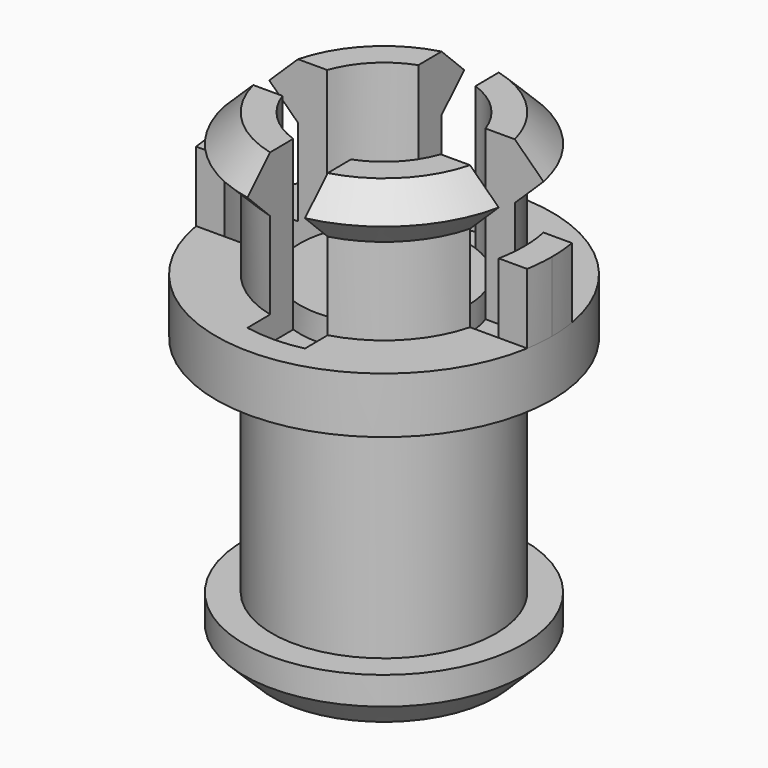
from build123d import *

# Parameters (mm, degrees)
F0_R      = 5
F1_DEPTH  = 2
F2_R      = 4
F3_DEPTH  = 8
F4_R      = 6
F5_DEPTH  = 2
F7_DEPTH  = 2.5
F10_DEPTH = 8
F11_SIZE  = 1
F8_R      = 4
F8_R_2    = 3
F12_DEPTH = 3.1
F13_R     = 5
F13_R_2   = 4
F13_R_3   = 3
F14_DEPTH = 2
F16_DEPTH = 6
F17_SIZE  = 0.99999


# Not quite as in the source:
# - a fillet or chamfer is up to 0.001 mm smaller than in the source, because OpenCascade refuses the exact size


with BuildPart() as f1:
    # F0 (on Top) → F1 (new body)
    with BuildSketch(Plane.XY):
        Circle(F0_R)
    extrude(amount=F1_DEPTH)

    # F2 (on face) → F3 (join)
    with BuildSketch(Plane.XY.offset(2)):
        Circle(F2_R)
    extrude(amount=F3_DEPTH)

    # F4 (on face) → F5 (join)
    with BuildSketch(Plane.XY.offset(10)):
        Circle(F4_R)
    extrude(amount=F5_DEPTH)

    # F6 (on face) → F7 (join)
    with BuildSketch(Plane.XY.offset(12)):
        with BuildLine():
            ThreePointArc((6, 0), (5.9789831367, 0.5017575617), (5.9160797831, 1))
            Line((5.9160797831, 1), (4.5160797831, 1))
            Line((4.5160797831, 1), (4.5160797831, -1))
            Line((4.5160797831, -1), (5.9160797831, -1))
            ThreePointArc((5.9160797831, -1), (5.9789831367, -0.5017575617), (6, 0))
        make_face()
        with BuildLine():
            Line((-4.5160797831, 1), (-5.9160797831, 1))
            ThreePointArc((-5.9160797831, 1), (-6, 0), (-5.9160797831, -1))
            Line((-5.9160797831, -1), (-4.5160797831, -1))
            Line((-4.5160797831, -1), (-4.5160797831, 1))
        make_face()
    extrude(amount=F7_DEPTH)

    # F9 (on face) → F10 (cut)
    with BuildSketch(Plane(origin=(0, 0, 0), x_dir=(1, 0, 0), z_dir=(0, 0, -1))):
        with BuildLine():
            ThreePointArc((1.6, 2.6), (0, 3.0528675045), (-1.6, 2.6))
            Line((-1.6, 2.6), (-1.6, -2.6))
            ThreePointArc((-1.6, -2.6), (0, -3.0528675045), (1.6, -2.6))
            Line((1.6, -2.6), (1.6, 2.6))
        make_face()
    extrude(amount=-F10_DEPTH, mode=Mode.SUBTRACT)

    # F11
    f11_edges = [f1.edges().sort_by_distance(p)[0] for p in [
        (-5, 0, 0),
    ]]
    chamfer(f11_edges, length=F11_SIZE)

    # F8 (on face) → F12 (join)
    with BuildSketch(Plane.XY.offset(12)):
        Circle(F8_R)
        Circle(F8_R_2, mode=Mode.SUBTRACT)
    extrude(amount=F12_DEPTH)

    # F13 (on face) → F14 (join)
    with BuildSketch(Plane.XY.offset(15.1)):
        Circle(F13_R)
        Circle(F13_R_2, mode=Mode.SUBTRACT)
        Circle(F13_R_2)
        Circle(F13_R_3, mode=Mode.SUBTRACT)
    extrude(amount=F14_DEPTH)

    # F15 (on face) → F16 (cut)
    with BuildSketch(Plane.XY.offset(17.1)):
        with BuildLine():
            Line((-2.8284271247, 1), (-4.8989794856, 1))
            ThreePointArc((-4.8989794856, 1), (-5, 0), (-4.8989794856, -1))
            Line((-4.8989794856, -1), (-2.8284271247, -1))
            ThreePointArc((-2.8284271247, -1), (-3, 0), (-2.8284271247, 1))
        make_face()
        with BuildLine():
            ThreePointArc((0.9908586892, 4.9008365672), (-0.0278443772, 4.9999224685), (-1.0453806817, 4.8894968279))
            Line((-1.0453806817, 4.8894968279), (-1.0261823806, 2.819033473))
            ThreePointArc((-1.0261823806, 2.819033473), (-0.0085441177, 2.999987833), (1.0101083624, 2.8248329324))
            Line((1.0101083624, 2.8248329324), (0.9908586892, 4.9008365672))
        make_face()
        with BuildLine():
            ThreePointArc((5, 0), (4.974680765, 0.50254481), (4.8989794856, 1))
            Line((4.8989794856, 1), (2.8284271247, 1))
            ThreePointArc((2.8284271247, 1), (2.956795679, 0.5073059362), (3, 0))
            ThreePointArc((3, 0), (2.956795679, -0.5073059362), (2.8284271247, -1))
            Line((2.8284271247, -1), (4.8989794856, -1))
            ThreePointArc((4.8989794856, -1), (4.974680765, -0.50254481), (5, 0))
        make_face()
        with BuildLine():
            Line((-0.9737316464, -2.8375776079), (-0.9545333452, -4.9080409628))
            ThreePointArc((-0.9545333452, -4.9080409628), (0.0648756616, -4.9995790971), (1.0815661863, -4.8816200779))
            Line((1.0815661863, -4.8816200779), (1.0623165131, -2.8056164431))
            ThreePointArc((1.0623165131, -2.8056164431), (0.0470871391, -2.9996304441), (-0.9737316464, -2.8375776079))
        make_face()
    extrude(amount=-F16_DEPTH, mode=Mode.SUBTRACT)

    # F17 (size 1 in the source; OpenCascade refuses exactly that, so slightly less here)
    f17_edges = [f1.edges().sort_by_distance(p)[0] for p in [
        (3.564895, -3.505927, 15.1),
        (-3.551887, 3.519105, 15.1),
        (-3.519105, -3.551887, 15.1),
        (3.564895, -3.505927, 17.1),
        (-3.519105, -3.551887, 17.1),
        (-3.551887, 3.519105, 17.1),
        (3.532234, 3.53883, 17.1),
        (3.532234, 3.53883, 15.1),
    ]]
    chamfer(f17_edges, length=F17_SIZE)


solid = f1.part
